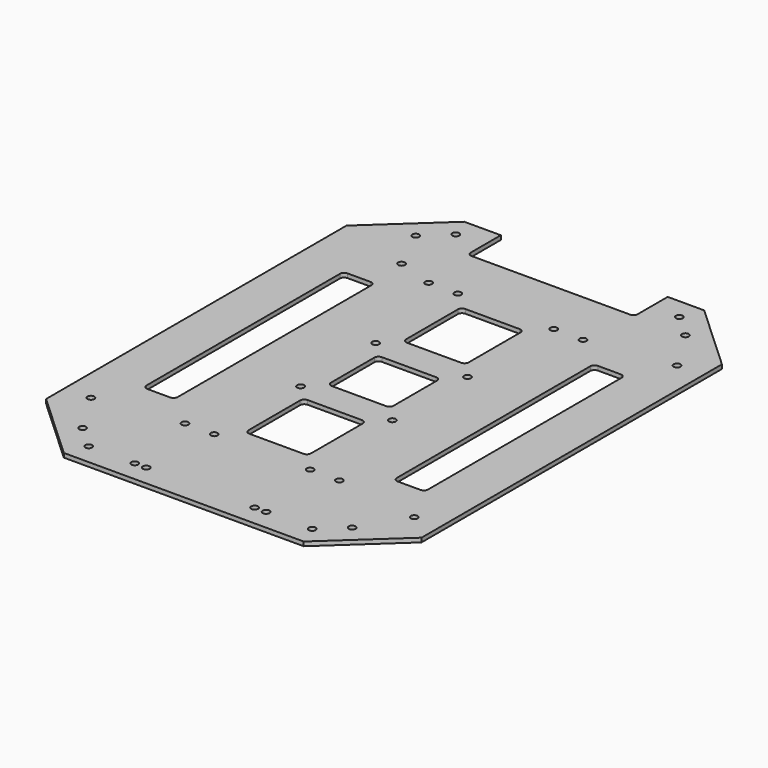
from build123d import *

# Parameters (mm, degrees)
F0_W     = 180
F0_H     = 180
F1_DEPTH = 2
F2_D     = 3.3
F4_D     = 3.3
F6_D     = 3.3
F7_W     = 30
F7_H     = 30
F7_H_2   = 35
F7_W_2   = 15
F7_H_3   = 120
F7_W_3   = 80
F7_H_4   = 20
F8_DEPTH = 2.001
F9_R     = 2


with BuildPart() as f1:
    # F0 (on Top) → F1 (new body)
    with BuildSketch(Plane.XY):
        Rectangle(F0_W, F0_H)
        Polygon((-90, 90), (90, 90), (57.5, 120), (-57.5, 120), align=None)
        Polygon((57.5, -120), (90, -90), (-90, -90), (-57.5, -120), align=None)
    extrude(amount=F1_DEPTH)

    # F2 (through all)
    with Locations(Plane(origin=(0, 0, 0), x_dir=(1, 0, 0), z_dir=(0, 0, -1))):
        with Locations((-23, -73), (23, -73), (23, 73), (-23, 73), (-54.58, -78.75), (37, -73), (77.5, -78.75), (-77.5, 78.75), (-37, 73), (77.5, 78.75), (37, 73), (-37, -73)):
            Hole(F2_D / 2)

    # F4 (through all)
    with Locations(Plane(origin=(0, 0, 0), x_dir=(1, 0, 0), z_dir=(0, 0, -1))):
        with Locations((-64.6122133253, 99.825798459), (-53.5901616559, 110), (53.5901616559, 110), (64.6122133253, 99.825798459), (64.6122133253, -99.825798459), (53.5901616559, -110), (-53.5901616559, -110), (-64.6122133253, -99.825798459)):
            Hole(F4_D / 2)

    # F6 (through all)
    with Locations(Plane(origin=(0, 0, 0), x_dir=(1, 0, 0), z_dir=(0, 0, -1))):
        with Locations((-22, -22.5), (22, -22.5), (22, 22.5), (-22, 22.5), (25.9754041397, 110), (31.4754041397, 110), (-25.9754041397, 110), (-31.4754041397, 110)):
            Hole(F6_D / 2)

    # F7 (on Top) → F8 (cut, through all)
    with BuildSketch(Plane.XY):
        Rectangle(F7_W, F7_H)
        with Locations((0, 47.5)):
            Rectangle(F7_W, F7_H_2)
        with Locations((0, -47)):
            Rectangle(F7_W, F7_H_2)
        with Locations((-60, 0)):
            Rectangle(F7_W_2, F7_H_3)
        with Locations((60, 0)):
            Rectangle(F7_W_2, F7_H_3)
        with Locations((0, 110)):
            Rectangle(F7_W_3, F7_H_4)
    extrude(amount=F8_DEPTH, mode=Mode.SUBTRACT)

    # F9
    f9_edges = [f1.edges().sort_by_distance(p)[0] for p in [
        (-52.5, -60, 1),
        (-67.5, -60, 1),
        (-52.5, 60, 1),
        (15, 65, 1),
        (15, 15, 1),
        (15, -29.5, 1),
        (67.5, 60, 1),
        (15, 30, 1),
        (15, -15, 1),
        (67.5, -60, 1),
        (40, 100, 1),
        (15, -64.5, 1),
        (-67.5, 60, 1),
        (-15, 65, 1),
        (-15, 15, 1),
        (-15, -29.5, 1),
        (52.5, -60, 1),
        (-15, -64.5, 1),
        (-40, 100, 1),
        (-15, -15, 1),
        (-15, 30, 1),
        (52.5, 60, 1),
    ]]
    fillet(f9_edges, radius=F9_R)


solid = f1.part
